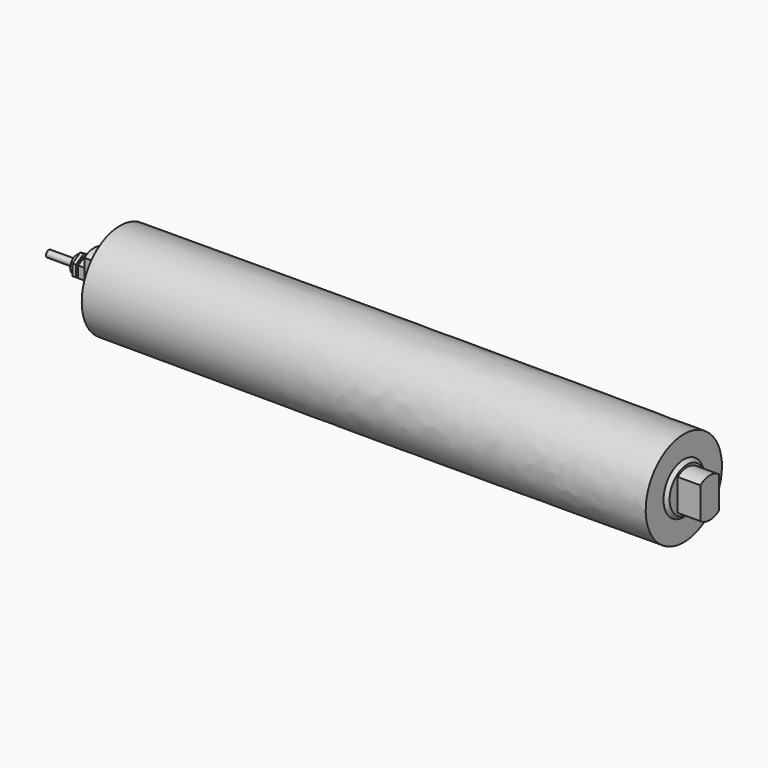
from build123d import *

# Parameters (mm, degrees)
F0_W      = 500
F0_H      = 42.25
F4_W      = 21
F4_H      = 28
F5_DEPTH  = 20
F7_DEPTH  = 15
F8_R      = 7.5
F9_DEPTH  = 3
F10_W     = 2
F10_H     = 2.5
F12_R     = 3
F13_DEPTH = 25


# Not quite as in the source:
# - a pattern or mirror of a feature is missing from the dataset's text; its kind, count and spacing are read off the source's solid


with BuildPart() as f1:
    # F0 (on Front) → F1 (revolve)
    with BuildSketch(Plane.XZ):
        with Locations((0, 21.125)):
            Rectangle(F0_W, F0_H)
        with BuildLine():
            ThreePointArc((250, 42.25), (0, 42.75), (-250, 42.25))
            Line((-250, 42.25), (250, 42.25))
        make_face()
    revolve(axis=Axis((0, 0, 0), (1, 0, 0)))

    # F2 (on Front) → F3 (revolve)
    with BuildSketch(Plane.XZ):
        Polygon((-253, 0), (-250, 0), (-250, 22.5), (-253, 19.5), align=None)
    f3 = revolve(axis=Axis((-251.5, 0, 0), (-1, 0, 0)))

    # F3_copies: F3 across plane
    add(f3.mirror(Plane(origin=(0, 0, 0), x_dir=(0, 0, 1), z_dir=(1, 0, 0))))

    # F4 (on face) → F5 (join)
    with BuildSketch(Plane(origin=(-253, 0, 0), x_dir=(0, -1, 0), z_dir=(-1, 0, 0))):
        Rectangle(F4_W, F4_H)
        with BuildLine():
            ThreePointArc((10.5, 14), (0, 17.5), (-10.5, 14))
            Line((-10.5, 14), (10.5, 14))
        make_face()
        with BuildLine():
            Line((10.5, -14), (-10.5, -14))
            ThreePointArc((-10.5, -14), (0, -17.5), (10.5, -14))
        make_face()
    f5 = extrude(amount=F5_DEPTH)

    # F5_copies: F5 across plane
    add(f5.mirror(Plane(origin=(0, 0, 0), x_dir=(0, 0, 1), z_dir=(1, 0, 0))))

    # F6 (on face) → F7 (join)
    with BuildSketch(Plane(origin=(-273, 0, 0), x_dir=(0, -1, 0), z_dir=(-1, 0, 0))):
        Polygon((0, 10), (-8.6602540378, 5), (-8.6602540378, -5), (0, -10), (8.6602540378, -5), (8.6602540378, 5), align=None)
    extrude(amount=F7_DEPTH)

    # F8 (on face) → F9 (cut)
    with BuildSketch(Plane(origin=(-288, 0, 0), x_dir=(0, -1, 0), z_dir=(-1, 0, 0))):
        Polygon((0, 10), (-8.6602540378, 5), (-8.6602540378, -5), (0, -10), (8.6602540378, -5), (8.6602540378, 5), align=None)
        Circle(F8_R, mode=Mode.SUBTRACT)
    extrude(amount=-F9_DEPTH, mode=Mode.SUBTRACT)

    # F10 (on Front) → F11 (revolve, cut)
    with BuildSketch(Plane.XZ):
        with Locations((-281, 8.75)):
            Rectangle(F10_W, F10_H)
    revolve(axis=Axis((-10, 0, 0), (-1, 0, 0)), mode=Mode.SUBTRACT)

    # F12 (on face) → F13 (join)
    with BuildSketch(Plane(origin=(-288, 0, 0), x_dir=(0, -1, 0), z_dir=(-1, 0, 0))):
        Circle(F12_R)
    extrude(amount=F13_DEPTH)


solid = f1.part
